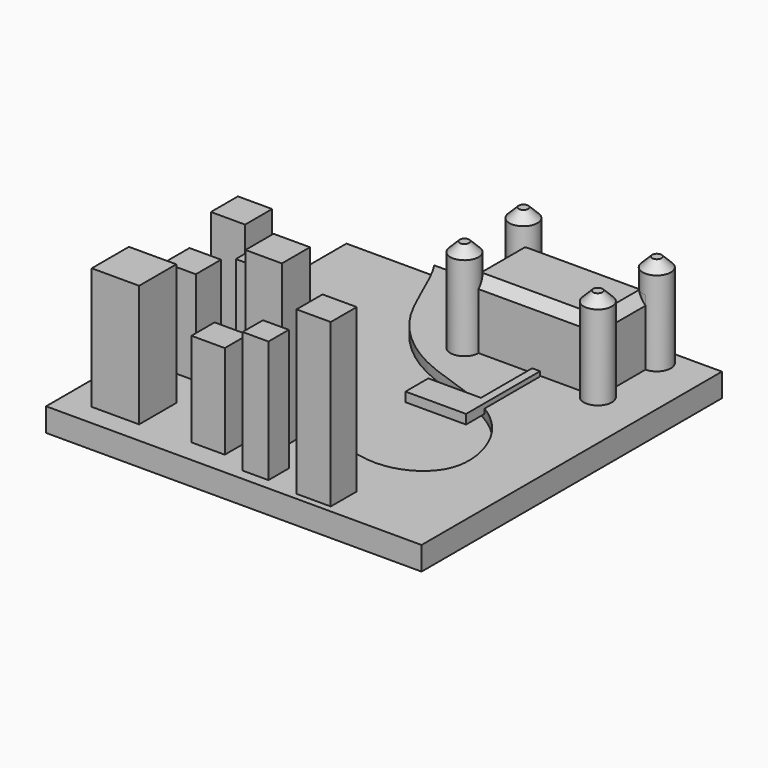
from build123d import *

# Parameters (mm, degrees)
F0_W          = 101.6
F0_H          = 101.6
F1_DEPTH      = 6.35
F3_DEPTH      = 2.54
F4_W          = 8.5470639169
F4_H          = 8.5470620543
F4_W_2        = 9.0218987316
F4_H_2        = 7.8348070383
F4_W_3        = 5.9354603291
F4_H_3        = 6.6477134824
F10_DEPTH     = 25.4
F5_W          = 9.2593189329
F5_H          = 9.1406079009
F5_W_2        = 8.5470620543
F5_H_2        = 9.2593189329
F5_W_3        = 12.8205921501
F5_H_3        = 12.5831738114
F5_W_4        = 7.0038423873
F5_H_4        = 6.885137409
F11_DEPTH     = 33.02
F6_W          = 9.8528647795
F6_H          = 9.4967372715
F6_W_2        = 9.2593152076
F6_H_2        = 8.7844803929
F12_DEPTH     = 43.942
F7_R          = 1.5202204641
F13_DEPTH     = 12.954
F8_W          = 36.0875949264
F8_H          = 19.9431441724
F14_DEPTH     = 17.78
F15_R         = 3.81
F16_DEPTH     = 25.4
F17_SIZE      = 2.54
F18_T4_DEPTH  = 25.3872937513
F18_S5_R      = 3.81
F18_T6_DEPTH  = 14
F18_S7_R      = 3.81
F18_T8_DEPTH  = 14
F18_T12_DEPTH = 41.5317445052
F18_S13_R     = 3.81
F18_T14_DEPTH = 22
F18_S15_R     = 3.81
F18_T16_DEPTH = 22
F18_T20_DEPTH = 25.3872937513
F18_S21_R     = 3.81
F18_T22_DEPTH = 14
F18_S23_R     = 3.81
F18_T24_DEPTH = 14
F18_T28_DEPTH = 41.5317445052
F18_S29_R     = 3.81
F18_T30_DEPTH = 22
F18_S31_R     = 3.81
F18_T32_DEPTH = 22
F9_W          = 14.245100785
F9_H          = 7.716097869
F19_DEPTH     = 1.27


# Not quite as in the source:
# - a fillet or chamfer that OpenCascade refuses, or shapes differently, is made with other operations: its cross-section is extruded or revolved along the edge and cut away or added


with BuildPart() as f1:
    # F0 (on Top) → F1 (new body)
    with BuildSketch(Plane.XY):
        Rectangle(F0_W, F0_H)
    extrude(amount=-F1_DEPTH)

    # F2 (on Top) → F3 (cut)
    with BuildSketch(Plane.XY):
        with BuildLine():
            add(Edge.make_bspline(
                [(-43.0914387107, 13.8889765367), (-48.792132623, 16.8713450612), (-60.3046561951, 22.7349998179), (-64.7610317916, 39.255042485), (-64.8154675332, 45.423523183)],
                knots=[0, 0, 0, 0, 0.4841794351, 1, 1, 1, 1], degree=3))
            add(Edge.make_bspline(
                [(-43.0914387107, 13.8889765367), (-37.3227409256, 12.4784266372), (-25.238481151, 9.5236064613), (-8.5238992218, -4.1081865608), (-5.0933643721, -15.7347262944), (10.2382263796, -27.360890695), (25.1611930237, -28.3877213638), (35.757581674, -20.0820321549), (33.8435161562, -4.7561465103), (22.6073453238, 8.7237537482), (-1.0459930134, 13.2625730637), (-18.464949103, 28.4069952294), (-24.7392805682, 51.2806449877), (-36.4483970668, 62.0438769385), (-40.598793265, 65.3666710807)],
                knots=[0, 0, 0, 0, 0.0857293443, 0.1753055598, 0.2440669449, 0.3285210308, 0.4037415508, 0.4706009031, 0.5439255605, 0.6247496782, 0.7209366486, 0.814216246, 0.9108692703, 1, 1, 1, 1], degree=3))
            Line((-40.598793265, 65.3666710807), (-64.8154675332, 45.423523183))
        make_face()
    extrude(amount=-F3_DEPTH, mode=Mode.SUBTRACT)

    # F4 (on Top) → F10 (join)
    with BuildSketch(Plane.XY):
        with Locations((-37.6308169216, -17.6876699552)):
            Rectangle(F4_W, F4_H)
        with Locations((-11.9896298274, -40.5985452235)):
            Rectangle(F4_W_2, F4_H_2)
        with Locations((13.5328508914, -33.3572849631)):
            Rectangle(F4_W_3, F4_H_3)
    extrude(amount=F10_DEPTH)

    # F5 (on Top) → F11 (join)
    with BuildSketch(Plane.XY):
        with Locations((-34.900506027, -4.5703039505)):
            Rectangle(F5_W, F5_H)
        with Locations((-17.6876718178, -18.0437983945)):
            Rectangle(F5_W_2, F5_H_2)
        with Locations((-36.6811426356, -38.6991985142)):
            Rectangle(F5_W_3, F5_H_3)
        with Locations((3.5019211937, -44.3972405046)):
            Rectangle(F5_W_4, F5_H_4)
    extrude(amount=F11_DEPTH)

    # F6 (on Top) → F12 (join)
    with BuildSketch(Plane.XY):
        with Locations((-4.9264323898, -29.7960098833)):
            Rectangle(F6_W, F6_H)
        with Locations((20.1805653051, -44.6346588433)):
            Rectangle(F6_W_2, F6_H_2)
    extrude(amount=F12_DEPTH)

    # F7 (on Top) → F13 (join)
    with BuildSketch(Plane.XY):
        with Locations((-21.7237845063, -2.0180563442)):
            Circle(F7_R)
    extrude(amount=F13_DEPTH)

    # F8 (on Top) → F14 (join)
    with BuildSketch(Plane.XY):
        with Locations((19.5870175958, 35.2566316724)):
            Rectangle(F8_W, F8_H)
    extrude(amount=F14_DEPTH)

    # F15 (on Top) → F16 (join)
    with BuildSketch(Plane.XY):
        with Locations((1.5432201326, 45.2282037586)):
            Circle(F15_R)
        with Locations((37.6308150589, 45.2282037586)):
            Circle(F15_R)
        with Locations((37.6308150589, 25.2850595862)):
            Circle(F15_R)
        with Locations((1.5432201326, 25.2850595862)):
            Circle(F15_R)
    extrude(amount=F16_DEPTH)

    # F17
    f17_edges = [f1.edges().sort_by_distance(p)[0] for p in [
        (-2.26678, 45.228204, 25.4),
        (-2.26678, 25.28506, 25.4),
        (33.820815, 25.28506, 25.4),
        (33.820815, 45.228204, 25.4),
    ]]
    chamfer(f17_edges, length=F17_SIZE)

    # F18: chamfer of 2.54 on 4 edges, made by hand


with BuildPart() as f18_tool2:
    # F18_s3 → F18_t4 (new body)
    with BuildSketch(Plane.XZ.offset(-47.950278548)):
        Polygon((4.0832201326, 17.78), (1.5432201326, 15.24), (1.5432201326, 17.78), align=None)
    extrude(amount=F18_T4_DEPTH)

    # F18_s5 → F18_t6 (cut, symmetric)
    with BuildSketch(Plane.XY.offset(16.5)):
        with Locations((1.5432201326, 25.2850595862)):
            Circle(F18_S5_R)
    extrude(amount=F18_T6_DEPTH, both=True, mode=Mode.SUBTRACT)

    # F18_s7 → F18_t8 (cut, symmetric)
    with BuildSketch(Plane.XY.offset(16.5)):
        with Locations((1.5432201326, 45.2282037586)):
            Circle(F18_S7_R)
    extrude(amount=F18_T8_DEPTH, both=True, mode=Mode.SUBTRACT)


with BuildPart() as f1_1:
    add(f1.part)

    # F18_t1: cut F18_tool2
    add(f18_tool2.part, mode=Mode.SUBTRACT)


with BuildPart() as f18_tool10:
    # F18_s11 → F18_t12 (new body)
    with BuildSketch(Plane.YZ.offset(-1.1788546568)):
        Polygon((25.2850595862, 15.24), (27.8250595862, 17.78), (25.2850595862, 17.78), align=None)
    extrude(amount=F18_T12_DEPTH)

    # F18_s13 → F18_t14 (cut, symmetric)
    with BuildSketch(Plane.XY.offset(16.5)):
        with Locations((37.6308150589, 25.2850595862)):
            Circle(F18_S13_R)
    extrude(amount=F18_T14_DEPTH, both=True, mode=Mode.SUBTRACT)

    # F18_s15 → F18_t16 (cut, symmetric)
    with BuildSketch(Plane.XY.offset(16.5)):
        with Locations((1.5432201326, 25.2850595862)):
            Circle(F18_S15_R)
    extrude(amount=F18_T16_DEPTH, both=True, mode=Mode.SUBTRACT)


with BuildPart() as f1_2:
    add(f1_1.part)

    # F18_t9: cut F18_tool10
    add(f18_tool10.part, mode=Mode.SUBTRACT)


with BuildPart() as f18_tool18:
    # F18_s19 → F18_t20 (new body)
    with BuildSketch(Plane.XZ.offset(-22.5629847967)):
        Polygon((35.0908150589, 17.78), (37.6308150589, 15.24), (37.6308150589, 17.78), align=None)
    extrude(amount=-F18_T20_DEPTH)

    # F18_s21 → F18_t22 (cut, symmetric)
    with BuildSketch(Plane.XY.offset(16.5)):
        with Locations((37.6308150589, 25.2850595862)):
            Circle(F18_S21_R)
    extrude(amount=F18_T22_DEPTH, both=True, mode=Mode.SUBTRACT)

    # F18_s23 → F18_t24 (cut, symmetric)
    with BuildSketch(Plane.XY.offset(16.5)):
        with Locations((37.6308150589, 45.2282037586)):
            Circle(F18_S23_R)
    extrude(amount=F18_T24_DEPTH, both=True, mode=Mode.SUBTRACT)


with BuildPart() as f1_3:
    add(f1_2.part)

    # F18_t17: cut F18_tool18
    add(f18_tool18.part, mode=Mode.SUBTRACT)


with BuildPart() as f18_tool26:
    # F18_s27 → F18_t28 (new body)
    with BuildSketch(Plane.YZ.offset(40.3528898484)):
        Polygon((42.6882037586, 17.78), (45.2282037586, 15.24), (45.2282037586, 17.78), align=None)
    extrude(amount=-F18_T28_DEPTH)

    # F18_s29 → F18_t30 (cut, symmetric)
    with BuildSketch(Plane.XY.offset(16.5)):
        with Locations((1.5432201326, 45.2282037586)):
            Circle(F18_S29_R)
    extrude(amount=F18_T30_DEPTH, both=True, mode=Mode.SUBTRACT)

    # F18_s31 → F18_t32 (cut, symmetric)
    with BuildSketch(Plane.XY.offset(16.5)):
        with Locations((37.6308150589, 45.2282037586)):
            Circle(F18_S31_R)
    extrude(amount=F18_T32_DEPTH, both=True, mode=Mode.SUBTRACT)


with BuildPart() as f1_4:
    add(f1_3.part)

    # F18_t25: cut F18_tool26
    add(f18_tool26.part, mode=Mode.SUBTRACT)

    # F9 (on Top) → F19 (join, symmetric)
    with BuildSketch(Plane.XY):
        Polygon((22.1986230463, 0), (22.1986230463, 25.0476412475), (20.0618524104, 25.0476412475), (20.0618524104, 7.716097869), (20.0618524104, 0), align=None)
        with Locations((12.9393020179, 3.8580489345)):
            Rectangle(F9_W, F9_H)
    extrude(amount=F19_DEPTH, both=True)


solid = f1_4.part
